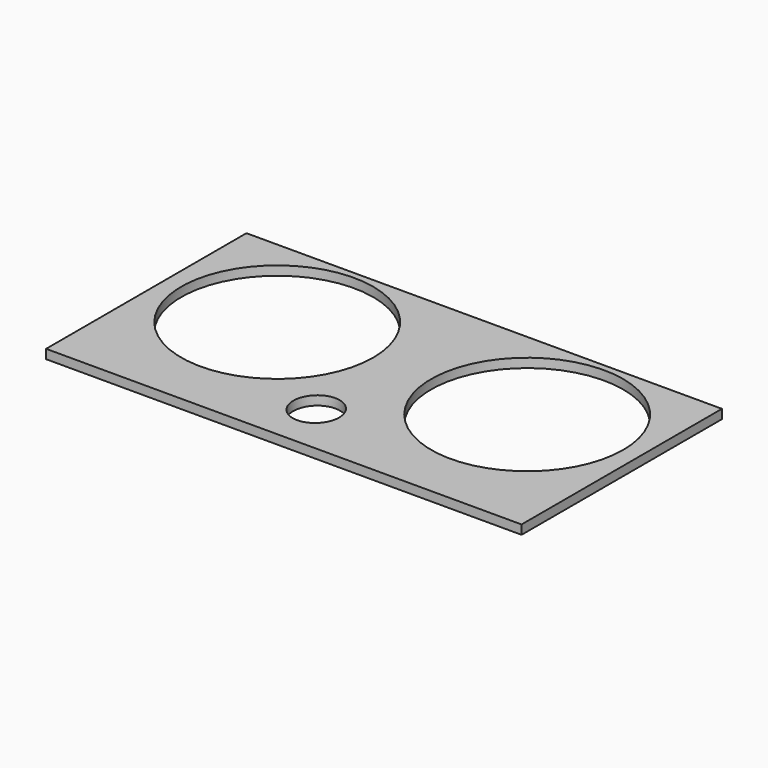
from build123d import *

# Parameters (mm, degrees)
F0_W     = 330.2
F0_H     = 173.9225888619
F0_R     = 66.675
F1_DEPTH = 6.35


# Not quite as in the source:
# - the dataset's text gives a spline's control points without its knots; the knots are read off the source's solid


with BuildPart() as f1:
    # F0 (on Top) → F1 (new body)
    with BuildSketch(Plane.XY):
        with Locations((-132.4583572531, -73.9906652679)):
            Rectangle(F0_W, F0_H)
        with BuildLine():
            add(Edge.make_bspline(
                [(-138.9201402808, -141.3304854369), (-138.3928185407, -141.3304854369), (-137.3381750605, -141.275400301), (-135.2625215798, -140.9492902881), (-133.2552416123, -140.3064688013), (-131.3632448334, -139.3625418043), (-129.5649193209, -138.2239224731), (-127.5612000685, -136.4834555233), (-125.9244832491, -134.3798930655), (-124.862585277, -132.5093025607), (-123.9869219901, -130.5516065921), (-123.3950651292, -128.4884227829), (-123.095646983, -126.3629935264), (-123.0198869297, -124.7450926538), (-123.095646983, -123.1271917812), (-123.3950651292, -121.0017625246), (-123.9869219901, -118.9385787154), (-124.862585277, -116.9808827469), (-125.9244832491, -115.110292242), (-127.5612000685, -113.0067297843), (-129.5649193209, -111.2662628345), (-131.3632448334, -110.1276435032), (-133.2552416123, -109.1837165063), (-135.2625215798, -108.5408950195), (-137.3381750605, -108.2147850066), (-138.9201402808, -108.1321573027), (-140.5021055011, -108.2147850066), (-142.5777589818, -108.5408950195), (-144.5850389493, -109.1837165063), (-146.4770357282, -110.1276435032), (-148.2753612407, -111.2662628345), (-150.2790804931, -113.0067297843), (-151.9157973125, -115.110292242), (-152.9776952845, -116.9808827469), (-153.8533585715, -118.9385787154), (-154.4452154324, -121.0017625246), (-154.7446335786, -123.1271917812), (-154.8203936319, -124.7450926538), (-154.7446335786, -126.3629935264), (-154.4452154324, -128.4884227829), (-153.8533585715, -130.5516065921), (-152.9776952845, -132.5093025607), (-151.9157973125, -134.3798930655), (-150.2790804931, -136.4834555233), (-148.2753612407, -138.2239224731), (-146.4770357282, -139.3625418043), (-144.5850389493, -140.3064688013), (-142.5777589818, -140.9492902881), (-140.5021055011, -141.275400301), (-139.4474620209, -141.3304854369), (-138.9201402808, -141.3304854369)],
                knots=[0, 0, 0, 0, 0.015625, 0.03125, 0.0625, 0.078125, 0.09375, 0.125, 0.15625, 0.171875, 0.1875, 0.21875, 0.234375, 0.25, 0.265625, 0.28125, 0.3125, 0.328125, 0.34375, 0.375, 0.40625, 0.421875, 0.4375, 0.46875, 0.484375, 0.5, 0.515625, 0.53125, 0.5625, 0.578125, 0.59375, 0.625, 0.65625, 0.671875, 0.6875, 0.71875, 0.734375, 0.75, 0.765625, 0.78125, 0.8125, 0.828125, 0.84375, 0.875, 0.90625, 0.921875, 0.9375, 0.96875, 0.984375, 1, 1, 1, 1], degree=3))
        make_face(mode=Mode.SUBTRACT)
        with Locations((-219.2488735842, -58.1939341619)):
            Circle(F0_R, mode=Mode.SUBTRACT)
        with Locations((-45.6678409221, -58.1939341619)):
            Circle(F0_R, mode=Mode.SUBTRACT)
    extrude(amount=F1_DEPTH)


solid = f1.part
